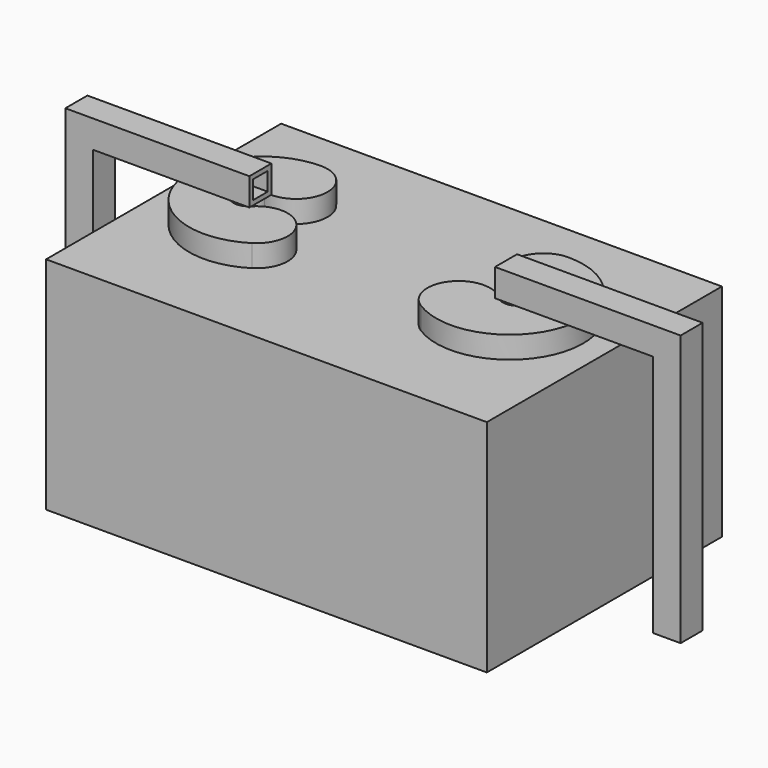
from build123d import *

# Parameters (mm, degrees)
F0_W     = 304.8
F0_H     = 152.4
F1_DEPTH = 203.2
F4_W     = 19.05
F4_H     = 19.05
F4_W_2   = 12.7
F4_H_2   = 12.7
F8_DEPTH = 15.24


with BuildPart() as f1:
    # F0 (on Front) → F1 (new body)
    with BuildSketch(Plane.XZ):
        with Locations((0, 76.2)):
            Rectangle(F0_W, F0_H)
    extrude(amount=-F1_DEPTH)


with BuildPart() as f5:
    # F5: sweep along a path in F3
    with BuildLine(Plane.XZ.offset(-101.6)) as f5_path:
        Line((203.2, 0), (203.2, 177.8))
        Line((203.2, 177.8), (84.3880101994, 177.8))
    # F4 (on Top) → F5 (sweep)
    with BuildSketch(Plane.XY):
        with Locations((203.2, 101.6)):
            Rectangle(F4_W, F4_H)
        with Locations((203.2, 101.6)):
            Rectangle(F4_W_2, F4_H_2, mode=Mode.SUBTRACT)
    sweep(path=f5_path.line, transition=Transition.RIGHT)


with BuildPart() as f6:
    # F6: sweep along a path in F3
    with BuildLine(Plane.XZ.offset(-101.6)) as f6_path:
        Line((-203.2, 0), (-203.2, 177.8))
        Line((-203.2, 177.8), (-85.4900650759, 177.8))
    # F4 (on Top) → F6 (sweep)
    with BuildSketch(Plane.XY):
        with Locations((-203.2, 101.6)):
            Rectangle(F4_W, F4_H)
        with Locations((-203.2, 101.6)):
            Rectangle(F4_W_2, F4_H_2, mode=Mode.SUBTRACT)
    sweep(path=f6_path.line, transition=Transition.RIGHT)

    # F7 (on face) → F8 (join)
    with BuildSketch(Plane(origin=(0, 0, 168.275), x_dir=(1, 0, 0), z_dir=(0, 0, -1))):
        with BuildLine():
            ThreePointArc((-58.4609373129, -60.3908278193), (-134.2912011879, -89.357700658), (-85.4743421078, -154.2131006718))
            ThreePointArc((-85.4743421078, -154.2131006718), (-63.9879107494, -130.0023087379), (-90.5800762449, -111.5446297711))
            ThreePointArc((-90.5800762449, -111.5446297711), (-103.2949896459, -98.2821615992), (-85.4743421078, -93.8115233757))
            ThreePointArc((-85.4743421078, -93.8115233757), (-53.1385123205, -92.3204531035), (-58.4609373129, -60.3908278193))
        make_face()
    extrude(amount=F8_DEPTH)


with BuildPart() as f8:
    # F7 (on face) → F8, piece 2 (new body)
    with BuildSketch(Plane(origin=(0, 0, 168.275), x_dir=(1, 0, 0), z_dir=(0, 0, -1))):
        with BuildLine():
            ThreePointArc((58.4609373129, -60.3908278193), (53.1385123205, -92.3204531035), (85.4743421078, -93.8115233757))
            ThreePointArc((85.4743421078, -93.8115233757), (103.2949896459, -98.2821615992), (90.5800762449, -111.5446297711))
            ThreePointArc((90.5800762449, -111.5446297711), (63.9879107494, -130.0023087379), (85.4743421078, -154.2131006718))
            ThreePointArc((85.4743421078, -154.2131006718), (134.2912011879, -89.357700658), (58.4609373129, -60.3908278193))
        make_face()
    extrude(amount=F8_DEPTH)


solid = Compound([f1.part, f5.part, f6.part, f8.part])
